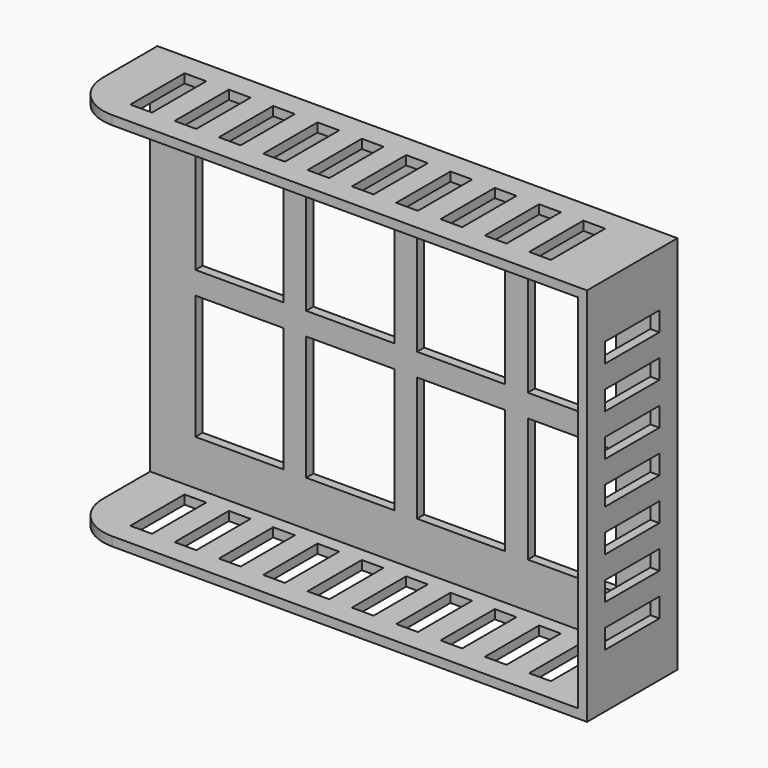
from build123d import *

# Parameters (mm, degrees)
F0_W     = 115
F0_H     = 84
F1_DEPTH = 25
F2_T     = -2
F3_R     = 10
F4_W     = 19.5
F4_H     = 27.5
F5_DEPTH = 25
F6_W     = 4.8
F6_H     = 15
F7_DEPTH = 84.001
F8_W     = 15
F8_H     = 4.286
F9_DEPTH = 25


with BuildPart() as f1:
    # F0 (on Front) → F1 (new body)
    with BuildSketch(Plane.XZ):
        with Locations((-91.9387002908, -17.9252284579)):
            Rectangle(F0_W, F0_H)
    extrude(amount=F1_DEPTH)

    # F2
    f2_openings = [f1.faces().sort_by_distance(p)[0] for p in [
        (-91.9387, -25, -17.925228),
        (-149.4387, -12.5, -17.925228),
    ]]
    offset(amount=F2_T, openings=f2_openings)

    # F3
    f3_edges = [f1.edges().sort_by_distance(p)[0] for p in [
        (-149.4387, -25, 23.074772),
        (-149.4387, -25, -58.925228),
    ]]
    fillet(f3_edges, radius=F3_R)

    # F4 (on face) → F5 (cut)
    with BuildSketch(Plane(origin=(0, 0, 0), x_dir=(-1, 0, 0), z_dir=(0, 1, 0))):
        with Locations((56.1887002908, -1.6752284579)):
            Rectangle(F4_W, F4_H)
        with Locations((80.6887002908, -1.6752284579)):
            Rectangle(F4_W, F4_H)
        with Locations((105.1887002908, -1.6752284579)):
            Rectangle(F4_W, F4_H)
        with Locations((129.6887002908, -1.6752284579)):
            Rectangle(F4_W, F4_H)
        with Locations((129.6887002908, -34.1752284579)):
            Rectangle(F4_W, F4_H)
        with Locations((105.1887002908, -34.1752284579)):
            Rectangle(F4_W, F4_H)
        with Locations((80.6887002908, -34.1752284579)):
            Rectangle(F4_W, F4_H)
        with Locations((56.1887002908, -34.1752284579)):
            Rectangle(F4_W, F4_H)
    extrude(amount=-F5_DEPTH, mode=Mode.SUBTRACT)

    # F6 (on face) → F7 (cut, through all)
    with BuildSketch(Plane.XY.offset(24.0747715421)):
        with Locations((-48.8387002908, -12.5)):
            Rectangle(F6_W, F6_H)
        with Locations((-58.6387002908, -12.5)):
            Rectangle(F6_W, F6_H)
        with Locations((-68.4387002908, -12.5)):
            Rectangle(F6_W, F6_H)
        with Locations((-78.2387002908, -12.5)):
            Rectangle(F6_W, F6_H)
        with Locations((-88.0387002908, -12.5)):
            Rectangle(F6_W, F6_H)
        with Locations((-97.8387002908, -12.5)):
            Rectangle(F6_W, F6_H)
        with Locations((-107.6387002908, -12.5)):
            Rectangle(F6_W, F6_H)
        with Locations((-117.4387002908, -12.5)):
            Rectangle(F6_W, F6_H)
        with Locations((-127.2387002908, -12.5)):
            Rectangle(F6_W, F6_H)
        with Locations((-137.0387002908, -12.5)):
            Rectangle(F6_W, F6_H)
    extrude(amount=-F7_DEPTH, mode=Mode.SUBTRACT)

    # F8 (on face) → F9 (cut)
    with BuildSketch(Plane.YZ.offset(-34.4387002908)):
        with Locations((-12.5, -45.7822284579)):
            Rectangle(F8_W, F8_H)
        with Locations((-12.5, -36.4965141579)):
            Rectangle(F8_W, F8_H)
        with Locations((-12.5, -27.2107998579)):
            Rectangle(F8_W, F8_H)
        with Locations((-12.5, -17.9250855579)):
            Rectangle(F8_W, F8_H)
        with Locations((-12.5, -8.6393712579)):
            Rectangle(F8_W, F8_H)
        with Locations((-12.5, 0.6463430421)):
            Rectangle(F8_W, F8_H)
        with Locations((-12.5, 9.9320573421)):
            Rectangle(F8_W, F8_H)
    extrude(amount=-F9_DEPTH, mode=Mode.SUBTRACT)


solid = f1.part
